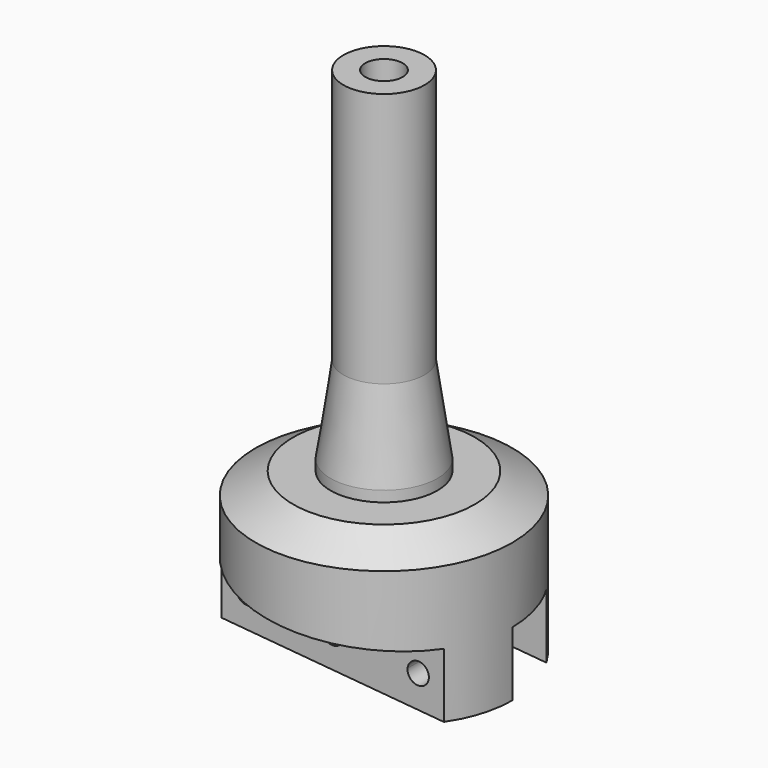
from build123d import *

# Parameters (mm, degrees)
F0_W     = 9.525
F0_H     = 50.8
F2_DEPTH = 38.1
F3_DEPTH = 19.05
F5_DEPTH = 19.05
F7_DEPTH = 19.05
F8_R     = 5.55625
F9_DEPTH = 31.75


with BuildPart() as f1:
    # F0 (on Front) → F1 (revolve)
    with BuildSketch(Plane.XZ):
        with Locations((4.7625, 25.4)):
            Rectangle(F0_W, F0_H)
        Polygon((0, 101.6), (0, 50.8), (9.525, 50.8), (9.525, 0), (15.875, 0), (12.0523, 25.8093433608), (12.0523, 101.6), align=None)
        Polygon((38.1, -31.4561230436), (0, -24.7380650786), (0, -28.3439140145), (38.1, -31.6772320948), align=None)
        Polygon((38.1, -31.6772320948), (0, -28.3439140145), (0, -44.081942035), (38.1, -50.8), align=None)
        Polygon((38.1, -50.8), (0, -44.081942035), (0, -47.4666819197), align=None)
        Polygon((38.1, -50.8), (0, -47.4666819197), (0, -50.8), align=None)
        Polygon((9.525, 0), (0, 0), (0, -24.7380650786), (38.1, -31.4561230436), (38.1, -9.5908048664), (26.9875, -3.175), (15.875, -3.175), (15.875, 0), align=None)
    revolve(axis=Axis((0, 0, -25.4), (0, 0, -1)))

    # F0 (on Front) → F2 (cut, symmetric)
    with BuildSketch(Plane.XZ):
        Polygon((0, -50.8), (0, -47.4666819197), (-38.1, -44.1333638393), (-38.1, -50.8), align=None)
        Polygon((38.1, -50.8), (0, -47.4666819197), (0, -50.8), align=None)
    extrude(amount=F2_DEPTH, both=True, mode=Mode.SUBTRACT)

    # F0 (on Front) → F3 (cut)
    with BuildSketch(Plane.XZ):
        Polygon((38.1, -31.6772320948), (0, -28.3439140145), (0, -44.081942035), (38.1, -50.8), align=None)
        Polygon((0, -44.081942035), (0, -28.3439140145), (-35.954874027, -25.1982701386), (-36.9244921743, -30.6972479093), (-37.5167449121, -37.4667276786), align=None)
        Polygon((0, -47.4666819197), (0, -44.081942035), (-37.5167449121, -37.4667276786), (-38.1, -44.1333638393), align=None)
        Polygon((38.1, -50.8), (0, -44.081942035), (0, -47.4666819197), align=None)
        Polygon((-36.9244921743, -30.6972479093), (-35.954874027, -25.1982701386), (-36.4396831007, -25.1558548407), align=None)
        Polygon((-38.1, -37.36388407), (-36.9244921743, -30.6972479093), (-36.4396831007, -25.1558548407), (-38.1, -25.0105959341), align=None)
        Polygon((-38.1, -37.36388407), (-37.5167449121, -37.4667276786), (-36.9244921743, -30.6972479093), align=None)
        Polygon((-38.1, -44.1333638393), (-37.5167449121, -37.4667276786), (-38.1, -37.36388407), align=None)
    extrude(amount=-F3_DEPTH, mode=Mode.SUBTRACT)

    # F4 (on face) → F5 (cut)
    with BuildSketch(Plane(origin=(-4.1212514076, 0, -47.106119142), x_dir=(0.9961946981, 0, -0.0871557427), z_dir=(-0.0871557427, 0, -0.9961946981))):
        with BuildLine():
            Line((-28.9846116747, 19.05), (4.5792120209, 19.05))
            Line((4.5792120209, 19.05), (37.2585995116, 19.05))
            add(Edge.make_bspline(
                [(4.1369939185, 38.1), (26.2180643139, 38.1), (37.2585995116, 19.05)],
                knots=[1.5707963268, 1.5707963268, 1.5707963268, 2.6058232788, 2.6058232788, 2.6058232788], degree=2, weights=[1, 0.8070072037, 0.8683475024]))
            add(Edge.make_bspline(
                [(-28.9846116747, 19.05), (-17.944076477, 38.1), (4.1369939185, 38.1)],
                knots=[0.5357693748, 0.5357693748, 0.5357693748, 1.5707963268, 1.5707963268, 1.5707963268], degree=2, weights=[0.8683475024, 0.8070072037, 1]))
        make_face()
        with BuildLine():
            Line((-34.1085418919, 19.05), (-28.9846116747, 19.05))
            add(Edge.make_bspline(
                [(-28.9846116747, 19.05), (-17.944076477, 38.1), (4.1369939185, 38.1)],
                knots=[0.5357693748, 0.5357693748, 0.5357693748, 1.5707963268, 1.5707963268, 1.5707963268], degree=2, weights=[0.8683475024, 0.8070072037, 1]))
            Line((4.1369939185, 38.1), (-34.1085418919, 38.1365224015))
            Line((-34.1085418919, 38.1365224015), (-34.1085418919, 19.05))
        make_face()
    extrude(amount=-F5_DEPTH, mode=Mode.SUBTRACT)

    # F6 (on face) → F7 (cut)
    with BuildSketch(Plane.XZ.offset(19.05)):
        with BuildLine():
            Line((3.1629181664, -38.1820174503), (-3.1629181664, -37.6285784838))
            ThreePointArc((-3.1629181664, -37.6285784838), (-0.2767194832, -41.0682161335), (3.1629181664, -38.1820174503))
        make_face()
        with BuildLine():
            ThreePointArc((3.175, -37.9052979671), (0.1384915549, -34.7333198635), (-3.1629181664, -37.6285784838))
            Line((-3.1629181664, -37.6285784838), (3.1629181664, -38.1820174503))
            ThreePointArc((3.1629181664, -38.1820174503), (3.1719781035, -38.0437895219), (3.175, -37.9052979671))
        make_face()
        with BuildLine():
            ThreePointArc((-22.225, -35.6830859135), (-25.2615084451, -32.51110781), (-28.5629181664, -35.4063664303))
            Line((-28.5629181664, -35.4063664303), (-22.2370818336, -35.9598053967))
            ThreePointArc((-22.2370818336, -35.9598053967), (-22.2280218965, -35.8215774684), (-22.225, -35.6830859135))
        make_face()
        with BuildLine():
            Line((-22.2370818336, -35.9598053967), (-28.5629181664, -35.4063664303))
            ThreePointArc((-28.5629181664, -35.4063664303), (-25.6767194832, -38.8460040799), (-22.2370818336, -35.9598053967))
        make_face()
        with BuildLine():
            ThreePointArc((22.2370818336, -39.8507905374), (25.1232805168, -43.2904281871), (28.5629181664, -40.4042295038))
            Line((28.5629181664, -40.4042295038), (22.2370818336, -39.8507905374))
        make_face()
        with BuildLine():
            Line((22.2370818336, -39.8507905374), (28.5629181664, -40.4042295038))
            ThreePointArc((28.5629181664, -40.4042295038), (28.5719781035, -40.2660015755), (28.575, -40.1275100206))
            ThreePointArc((28.575, -40.1275100206), (25.5384915549, -36.9555319171), (22.2370818336, -39.8507905374))
        make_face()
    extrude(amount=-F7_DEPTH, mode=Mode.SUBTRACT)

    # F8 (on face) → F9 (cut)
    with BuildSketch(Plane.XY.offset(101.6)):
        Circle(F8_R)
    extrude(amount=-F9_DEPTH, mode=Mode.SUBTRACT)


solid = f1.part
